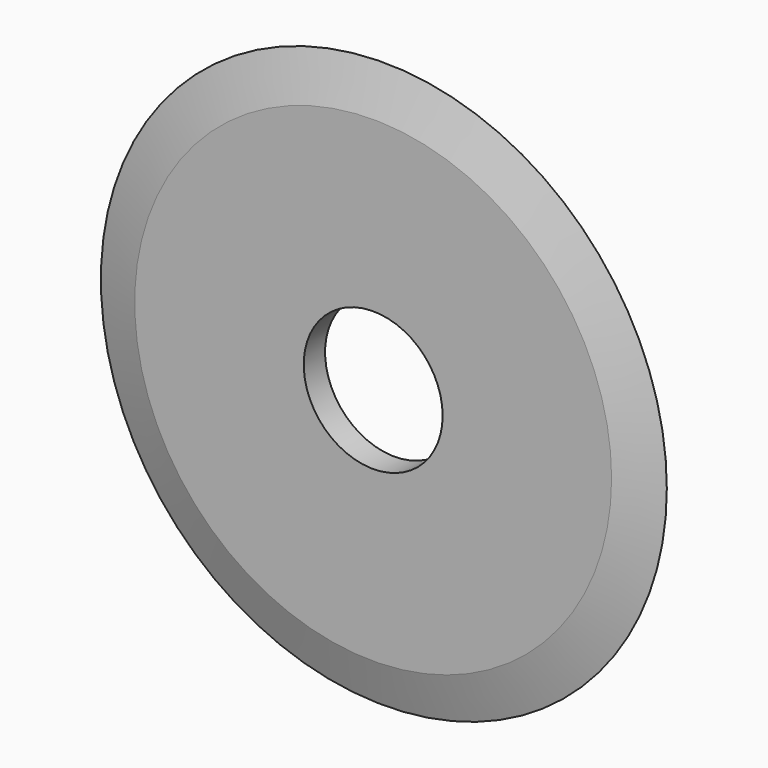
from build123d import *

# Parameters (mm, degrees)
F0_R     = 63.5490879023
F0_R_2   = 15.5969700922
F1_DEPTH = 3
F2_SIZE2 = 9.99999
F2_SIZE  = 2.99999


# Not quite as in the source:
# - a fillet or chamfer is up to 0.001 mm smaller than in the source, because OpenCascade refuses the exact size


with BuildPart() as f1:
    # F0 (on Front) → F1 (new body, symmetric)
    with BuildSketch(Plane.XZ):
        Circle(F0_R)
        Circle(F0_R_2, mode=Mode.SUBTRACT)
    extrude(amount=F1_DEPTH, both=True)

    # F2 (size 3 and 10 in the source; OpenCascade refuses exactly that, so slightly less here)
    f2_edges = [f1.edges().sort_by_distance(p)[0] for p in [
        (-63.549088, -3, 0),
        (-63.549088, 3, 0),
    ]]
    f2_side = f1.faces().sort_by_distance((-63.549088, 0, 0))[0]
    chamfer(f2_edges, length=F2_SIZE, length2=F2_SIZE2, reference=f2_side)


solid = f1.part
